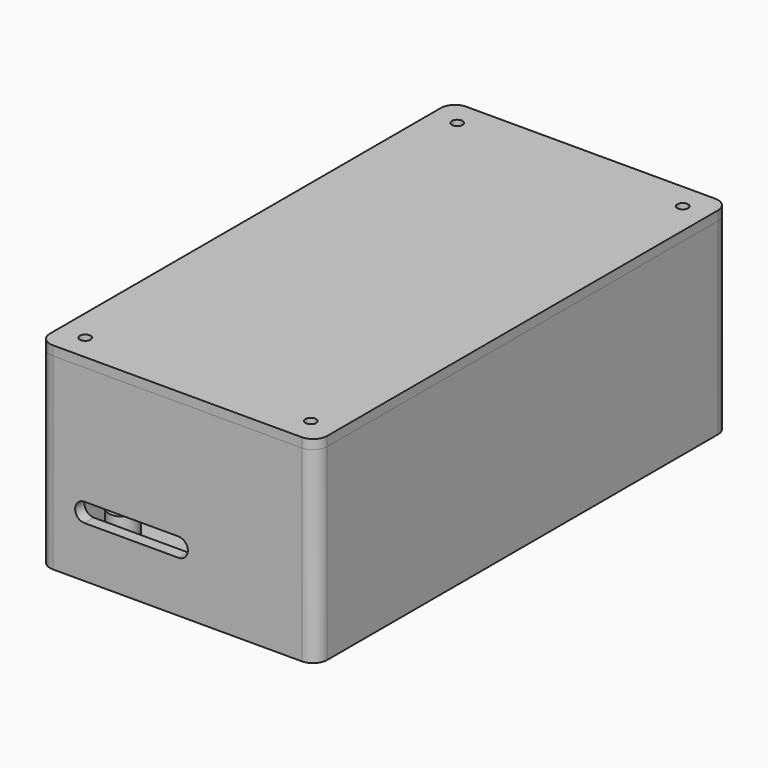
from build123d import *

# Parameters (mm, degrees)
F1_DEPTH  = 2
F2_DEPTH  = 38
F4_DEPTH  = 25
F6_DEPTH  = 25
F7_R      = 3
F7_R_2    = 1.25
F8_DEPTH  = 5.5
F10_DEPTH = 2.5
F11_DEPTH = 2
F12_R     = 1.55
F13_DEPTH = 120.8
F15_START = -3
F14_R     = 1.15
F15_DEPTH = 3
F16_R     = 1.15
F17_DEPTH = 25


with BuildPart() as f1:
    # F0 (on Top) → F1 (new body)
    with BuildSketch(Plane.XY):
        with BuildLine():
            Line((5.0090045333, 23.9092581272), (-47.9909954667, 23.9092581272))
            ThreePointArc((-47.9909954667, 23.9092581272), (-50.1123158103, 23.0305784708), (-50.9909954667, 20.9092581272))
            Line((-50.9909954667, 20.9092581272), (-50.9909954667, -83.0907418728))
            ThreePointArc((-50.9909954667, -83.0907418728), (-50.1123158103, -85.2120622163), (-47.9909954667, -86.0907418728))
            Line((-47.9909954667, -86.0907418728), (5.0090045333, -86.0907418728))
            ThreePointArc((5.0090045333, -86.0907418728), (7.1303248769, -85.2120622163), (8.0090045333, -83.0907418728))
            Line((8.0090045333, -83.0907418728), (8.0090045333, 20.9092581272))
            ThreePointArc((8.0090045333, 20.9092581272), (7.1303248769, 23.0305784708), (5.0090045333, 23.9092581272))
        make_face()
        with BuildLine():
            ThreePointArc((-48.4909954667, 18.4092581272), (-47.6123158103, 20.5305784708), (-45.4909954667, 21.4092581272))
            Line((-45.4909954667, 21.4092581272), (2.5090045333, 21.4092581272))
            ThreePointArc((2.5090045333, 21.4092581272), (4.6303248769, 20.5305784708), (5.5090045333, 18.4092581272))
            Line((5.5090045333, 18.4092581272), (5.5090045333, -80.5907418728))
            ThreePointArc((5.5090045333, -80.5907418728), (4.6303248769, -82.7120622163), (2.5090045333, -83.5907418728))
            Line((2.5090045333, -83.5907418728), (-45.4909954667, -83.5907418728))
            ThreePointArc((-45.4909954667, -83.5907418728), (-47.6123158103, -82.7120622163), (-48.4909954667, -80.5907418728))
            Line((-48.4909954667, -80.5907418728), (-48.4909954667, 18.4092581272))
        make_face(mode=Mode.SUBTRACT)
        with BuildLine():
            Line((2.5090045333, 21.4092581272), (-45.4909954667, 21.4092581272))
            ThreePointArc((-45.4909954667, 21.4092581272), (-47.6123158103, 20.5305784708), (-48.4909954667, 18.4092581272))
            Line((-48.4909954667, 18.4092581272), (-48.4909954667, -80.5907418728))
            ThreePointArc((-48.4909954667, -80.5907418728), (-47.6123158103, -82.7120622163), (-45.4909954667, -83.5907418728))
            Line((-45.4909954667, -83.5907418728), (2.5090045333, -83.5907418728))
            ThreePointArc((2.5090045333, -83.5907418728), (4.6303248769, -82.7120622163), (5.5090045333, -80.5907418728))
            Line((5.5090045333, -80.5907418728), (5.5090045333, 18.4092581272))
            ThreePointArc((5.5090045333, 18.4092581272), (4.6303248769, 20.5305784708), (2.5090045333, 21.4092581272))
        make_face()
    extrude(amount=-F1_DEPTH)

    # F0 (on Top) → F2 (join)
    with BuildSketch(Plane.XY):
        with BuildLine():
            Line((5.0090045333, 23.9092581272), (-47.9909954667, 23.9092581272))
            ThreePointArc((-47.9909954667, 23.9092581272), (-50.1123158103, 23.0305784708), (-50.9909954667, 20.9092581272))
            Line((-50.9909954667, 20.9092581272), (-50.9909954667, -83.0907418728))
            ThreePointArc((-50.9909954667, -83.0907418728), (-50.1123158103, -85.2120622163), (-47.9909954667, -86.0907418728))
            Line((-47.9909954667, -86.0907418728), (5.0090045333, -86.0907418728))
            ThreePointArc((5.0090045333, -86.0907418728), (7.1303248769, -85.2120622163), (8.0090045333, -83.0907418728))
            Line((8.0090045333, -83.0907418728), (8.0090045333, 20.9092581272))
            ThreePointArc((8.0090045333, 20.9092581272), (7.1303248769, 23.0305784708), (5.0090045333, 23.9092581272))
        make_face()
        with BuildLine():
            ThreePointArc((-48.4909954667, 18.4092581272), (-47.6123158103, 20.5305784708), (-45.4909954667, 21.4092581272))
            Line((-45.4909954667, 21.4092581272), (2.5090045333, 21.4092581272))
            ThreePointArc((2.5090045333, 21.4092581272), (4.6303248769, 20.5305784708), (5.5090045333, 18.4092581272))
            Line((5.5090045333, 18.4092581272), (5.5090045333, -80.5907418728))
            ThreePointArc((5.5090045333, -80.5907418728), (4.6303248769, -82.7120622163), (2.5090045333, -83.5907418728))
            Line((2.5090045333, -83.5907418728), (-45.4909954667, -83.5907418728))
            ThreePointArc((-45.4909954667, -83.5907418728), (-47.6123158103, -82.7120622163), (-48.4909954667, -80.5907418728))
            Line((-48.4909954667, -80.5907418728), (-48.4909954667, 18.4092581272))
        make_face(mode=Mode.SUBTRACT)
    extrude(amount=F2_DEPTH)

    # F3 (on face) → F4 (cut)
    with BuildSketch(Plane.XZ.offset(86.0907418728)):
        with BuildLine():
            ThreePointArc((-41.2469804287, 12.8703803271), (-43.2469804287, 10.8703803271), (-41.2469804287, 8.8703803271))
            Line((-41.2469804287, 8.8703803271), (-21.2469804287, 8.8703803271))
            ThreePointArc((-21.2469804287, 8.8703803271), (-19.2469804287, 10.8703803271), (-21.2469804287, 12.8703803271))
            Line((-21.2469804287, 12.8703803271), (-41.2469804287, 12.8703803271))
        make_face()
    extrude(amount=-F4_DEPTH, mode=Mode.SUBTRACT)

    # F5 (on face) → F6 (cut)
    with BuildSketch(Plane(origin=(0, 23.9092581272, 0), x_dir=(-1, 0, 0), z_dir=(0, 1, 0))):
        with BuildLine():
            ThreePointArc((6.3463230617, 13.4676470682), (3.0963230617, 10.2176470682), (6.3463230617, 6.9676470682))
            Line((6.3463230617, 6.9676470682), (26.636030525, 6.9676470682))
            ThreePointArc((26.636030525, 6.9676470682), (29.886030525, 10.2176470682), (26.636030525, 13.4676470682))
            Line((26.636030525, 13.4676470682), (6.3463230617, 13.4676470682))
        make_face()
    extrude(amount=-F6_DEPTH, mode=Mode.SUBTRACT)

    # F7 (on face) → F8 (join)
    with BuildSketch(Plane.XY):
        with Locations((-43.6000041664, 12.0808156207)):
            Circle(F7_R)
        with Locations((-43.6000041664, 12.0808156207)):
            Circle(F7_R_2, mode=Mode.SUBTRACT)
        with Locations((1.3999958336, 12.0808156207)):
            Circle(F7_R)
        with Locations((1.3999958336, 12.0808156207)):
            Circle(F7_R_2, mode=Mode.SUBTRACT)
        with Locations((-43.6000041664, -72.9191843793)):
            Circle(F7_R)
        with Locations((-43.6000041664, -72.9191843793)):
            Circle(F7_R_2, mode=Mode.SUBTRACT)
        with Locations((1.3999958336, -72.9191843793)):
            Circle(F7_R)
        with Locations((1.3999958336, -72.9191843793)):
            Circle(F7_R_2, mode=Mode.SUBTRACT)
    extrude(amount=F8_DEPTH)

    # F12 (on face) → F13 (cut)
    with BuildSketch(Plane.XY.offset(38)):
        with Locations((-31.9152586162, 15.2332521975)):
            Circle(F12_R)
        with Locations((-9.5154764131, 15.2332521975)):
            Circle(F12_R)
        with Locations((-31.9152586162, -72.9831755161)):
            Circle(F12_R)
        with Locations((-9.5154764131, -72.9831755161)):
            Circle(F12_R)
    extrude(amount=-F13_DEPTH, mode=Mode.SUBTRACT)

    # F14 (on face) → F15 (join)
    with BuildSketch(Plane.XY.offset(38).offset(F15_START)):
        with BuildLine():
            ThreePointArc((5.5090045333, -80.044771904), (0.3358921571, -78.5195149033), (2.1716910566, -83.5907418728))
            Line((2.1716910566, -83.5907418728), (2.5090045333, -83.5907418728))
            ThreePointArc((2.5090045333, -83.5907418728), (4.6303248769, -82.7120622163), (5.5090045333, -80.5907418728))
            Line((5.5090045333, -80.5907418728), (5.5090045333, -80.044771904))
        make_face()
        with Locations((2.5366169866, -80.5907418728)):
            Circle(F14_R, mode=Mode.SUBTRACT)
        with BuildLine():
            Line((-48.4909954667, -80.3297658185), (-48.4909954667, -80.5907418728))
            ThreePointArc((-48.4909954667, -80.5907418728), (-47.6123158103, -82.7120622163), (-45.4909954667, -83.5907418728))
            Line((-45.4909954667, -83.5907418728), (-45.2300194124, -83.5907418728))
            ThreePointArc((-45.2300194124, -83.5907418728), (-43.2713115333, -82.6257140438), (-42.4796654448, -80.5907418728))
            ThreePointArc((-42.4796654448, -80.5907418728), (-45.360384527, -77.5822456898), (-48.4909954667, -80.3297658185))
        make_face()
        with Locations((-45.4909954667, -80.5907418728)):
            Circle(F14_R, mode=Mode.SUBTRACT)
        with BuildLine():
            ThreePointArc((-45.4909954667, 21.4092581272), (-47.6123158103, 20.5305784708), (-48.4909954667, 18.4092581272))
            ThreePointArc((-48.4909954667, 18.4092581272), (-45.4909954667, 15.4092581272), (-42.4909954667, 18.4092581272))
            ThreePointArc((-42.4909954667, 18.4092581272), (-43.3696751231, 20.5305784708), (-45.4909954667, 21.4092581272))
        make_face()
        with Locations((-45.4909954667, 18.4092581272)):
            Circle(F14_R, mode=Mode.SUBTRACT)
        with BuildLine():
            Line((2.5090045333, 21.4092581272), (2.1279002239, 21.4092581272))
            ThreePointArc((2.1279002239, 21.4092581272), (0.3706359385, 16.2708895324), (5.5090045333, 18.0281538178))
            Line((5.5090045333, 18.0281538178), (5.5090045333, 18.4092581272))
            ThreePointArc((5.5090045333, 18.4092581272), (4.6303248769, 20.5305784708), (2.5090045333, 21.4092581272))
        make_face()
        with Locations((2.5090045333, 18.4092581272)):
            Circle(F14_R, mode=Mode.SUBTRACT)
    extrude(amount=-F15_DEPTH)


with BuildPart() as f10:
    # F9 (on face) → F10 (new body)
    with BuildSketch(Plane.XY.offset(38)):
        with BuildLine():
            Line((2.5090045333, 21.1092581272), (-45.4909954667, 21.1092581272))
            ThreePointArc((-45.4909954667, 21.1092581272), (-47.4001837759, 20.3184464364), (-48.1909954667, 18.4092581272))
            Line((-48.1909954667, 18.4092581272), (-48.1909954667, -80.5907418728))
            ThreePointArc((-48.1909954667, -80.5907418728), (-47.4001837759, -82.499930182), (-45.4909954667, -83.2907418728))
            Line((-45.4909954667, -83.2907418728), (2.5090045333, -83.2907418728))
            ThreePointArc((2.5090045333, -83.2907418728), (4.4181928425, -82.499930182), (5.2090045333, -80.5907418728))
            Line((5.2090045333, -80.5907418728), (5.2090045333, 18.4092581272))
            ThreePointArc((5.2090045333, 18.4092581272), (4.4181928425, 20.3184464364), (2.5090045333, 21.1092581272))
        make_face()
    extrude(amount=-F10_DEPTH)

    # F9 (on face) → F11 (join)
    with BuildSketch(Plane.XY.offset(38)):
        with BuildLine():
            Line((-50.9909954667, 20.9092581272), (-50.9909954667, -83.0907418728))
            ThreePointArc((-50.9909954667, -83.0907418728), (-50.1123158103, -85.2120622163), (-47.9909954667, -86.0907418728))
            Line((-47.9909954667, -86.0907418728), (5.0090045333, -86.0907418728))
            ThreePointArc((5.0090045333, -86.0907418728), (7.1303248769, -85.2120622163), (8.0090045333, -83.0907418728))
            Line((8.0090045333, -83.0907418728), (8.0090045333, 20.9092581272))
            ThreePointArc((8.0090045333, 20.9092581272), (7.1303248769, 23.0305784708), (5.0090045333, 23.9092581272))
            Line((5.0090045333, 23.9092581272), (-47.9909954667, 23.9092581272))
            ThreePointArc((-47.9909954667, 23.9092581272), (-50.1123158103, 23.0305784708), (-50.9909954667, 20.9092581272))
        make_face()
        with BuildLine():
            Line((-48.4909954667, -80.5907418728), (-48.4909954667, 18.4092581272))
            ThreePointArc((-48.4909954667, 18.4092581272), (-47.6123158103, 20.5305784708), (-45.4909954667, 21.4092581272))
            Line((-45.4909954667, 21.4092581272), (2.5090045333, 21.4092581272))
            ThreePointArc((2.5090045333, 21.4092581272), (4.6303248769, 20.5305784708), (5.5090045333, 18.4092581272))
            Line((5.5090045333, 18.4092581272), (5.5090045333, -80.5907418728))
            ThreePointArc((5.5090045333, -80.5907418728), (4.6303248769, -82.7120622163), (2.5090045333, -83.5907418728))
            Line((2.5090045333, -83.5907418728), (-45.4909954667, -83.5907418728))
            ThreePointArc((-45.4909954667, -83.5907418728), (-47.6123158103, -82.7120622163), (-48.4909954667, -80.5907418728))
        make_face(mode=Mode.SUBTRACT)
        with BuildLine():
            ThreePointArc((-45.4909954667, 21.4092581272), (-47.6123158103, 20.5305784708), (-48.4909954667, 18.4092581272))
            Line((-48.4909954667, 18.4092581272), (-48.4909954667, -80.5907418728))
            ThreePointArc((-48.4909954667, -80.5907418728), (-47.6123158103, -82.7120622163), (-45.4909954667, -83.5907418728))
            Line((-45.4909954667, -83.5907418728), (2.5090045333, -83.5907418728))
            ThreePointArc((2.5090045333, -83.5907418728), (4.6303248769, -82.7120622163), (5.5090045333, -80.5907418728))
            Line((5.5090045333, -80.5907418728), (5.5090045333, 18.4092581272))
            ThreePointArc((5.5090045333, 18.4092581272), (4.6303248769, 20.5305784708), (2.5090045333, 21.4092581272))
            Line((2.5090045333, 21.4092581272), (-45.4909954667, 21.4092581272))
        make_face()
        with BuildLine():
            ThreePointArc((-48.1909954667, 18.4092581272), (-47.4001837759, 20.3184464364), (-45.4909954667, 21.1092581272))
            Line((-45.4909954667, 21.1092581272), (2.5090045333, 21.1092581272))
            ThreePointArc((2.5090045333, 21.1092581272), (4.4181928425, 20.3184464364), (5.2090045333, 18.4092581272))
            Line((5.2090045333, 18.4092581272), (5.2090045333, -80.5907418728))
            ThreePointArc((5.2090045333, -80.5907418728), (4.4181928425, -82.499930182), (2.5090045333, -83.2907418728))
            Line((2.5090045333, -83.2907418728), (-45.4909954667, -83.2907418728))
            ThreePointArc((-45.4909954667, -83.2907418728), (-47.4001837759, -82.499930182), (-48.1909954667, -80.5907418728))
            Line((-48.1909954667, -80.5907418728), (-48.1909954667, 18.4092581272))
        make_face(mode=Mode.SUBTRACT)
        with BuildLine():
            Line((2.5090045333, 21.1092581272), (-45.4909954667, 21.1092581272))
            ThreePointArc((-45.4909954667, 21.1092581272), (-47.4001837759, 20.3184464364), (-48.1909954667, 18.4092581272))
            Line((-48.1909954667, 18.4092581272), (-48.1909954667, -80.5907418728))
            ThreePointArc((-48.1909954667, -80.5907418728), (-47.4001837759, -82.499930182), (-45.4909954667, -83.2907418728))
            Line((-45.4909954667, -83.2907418728), (2.5090045333, -83.2907418728))
            ThreePointArc((2.5090045333, -83.2907418728), (4.4181928425, -82.499930182), (5.2090045333, -80.5907418728))
            Line((5.2090045333, -80.5907418728), (5.2090045333, 18.4092581272))
            ThreePointArc((5.2090045333, 18.4092581272), (4.4181928425, 20.3184464364), (2.5090045333, 21.1092581272))
        make_face()
    extrude(amount=F11_DEPTH)

    # F16 (on face) → F17 (cut)
    with BuildSketch(Plane.XY.offset(40)):
        with Locations((2.5366169866, -80.5907418728)):
            Circle(F16_R)
        with Locations((-45.4909954667, -80.5907418728)):
            Circle(F16_R)
        with Locations((2.5090045333, 18.4092581272)):
            Circle(F16_R)
        with Locations((-45.4909954667, 18.4092581272)):
            Circle(F16_R)
    extrude(amount=-F17_DEPTH, mode=Mode.SUBTRACT)


solid = Compound([f1.part, f10.part])
